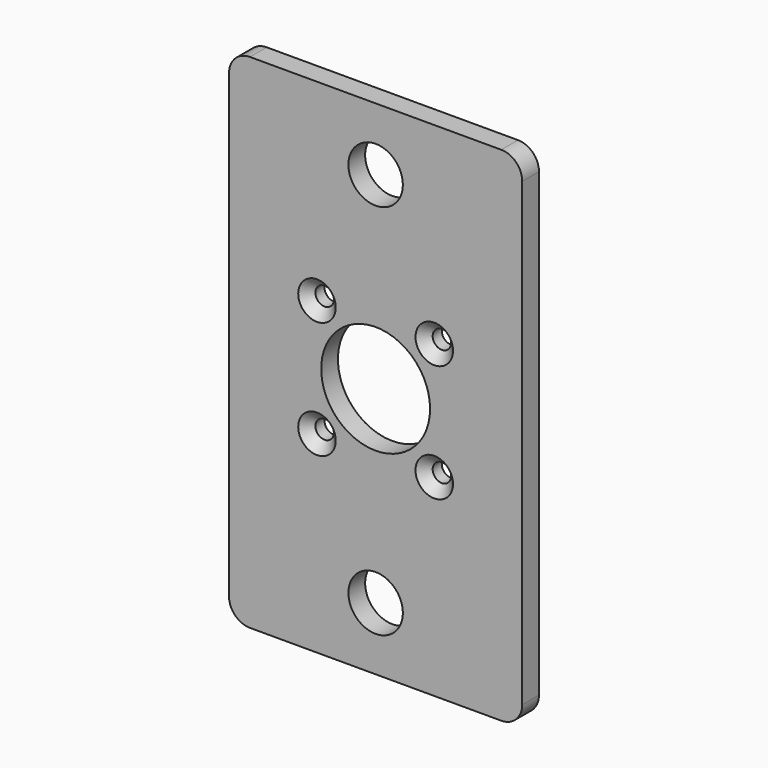
from build123d import *

# Parameters (mm, degrees)
F0_W           = 70
F0_H           = 120
F0_R           = 6.5
F0_R_2         = 13
F1_DEPTH       = 5
F3_D           = 4.4
F3_DEPTH       = 10
F3_CSINK_D     = 8.96
F3_CSINK_ANGLE = 90
F3_TIP         = 1.3218933619
F4_R           = 5


# Not quite as in the source:
# - a feature names something its author has since deleted; it is built from what else it names


with BuildPart() as f1:
    # F0 (on Front) → F1 (new body)
    with BuildSketch(Plane.XZ):
        Rectangle(F0_W, F0_H)
        with Locations((0, -45)):
            Circle(F0_R, mode=Mode.SUBTRACT)
        Circle(F0_R_2, mode=Mode.SUBTRACT)
        with Locations((0, 45)):
            Circle(F0_R, mode=Mode.SUBTRACT)
    extrude(amount=F1_DEPTH)

    # F3
    with Locations(Plane.XZ.offset(5)):
        with Locations((14, 14), (-14, 14), (-14, -14), (14, -14)):
            CounterSinkHole(F3_D / 2, F3_CSINK_D / 2, depth=F3_DEPTH, counter_sink_angle=F3_CSINK_ANGLE)
            with Locations((0, 0, -(F3_DEPTH + F3_TIP / 2))):  # 118° drill point
                Cone(0, F3_D / 2, F3_TIP, mode=Mode.SUBTRACT)

    # F4
    f4_edges = [f1.edges().sort_by_distance(p)[0] for p in [
        (35, -2.5, 60),
        (35, -2.5, -60),
        (-35, -2.5, -60),
        (-35, -2.5, 60),
    ]]
    fillet(f4_edges, radius=F4_R)


solid = f1.part
